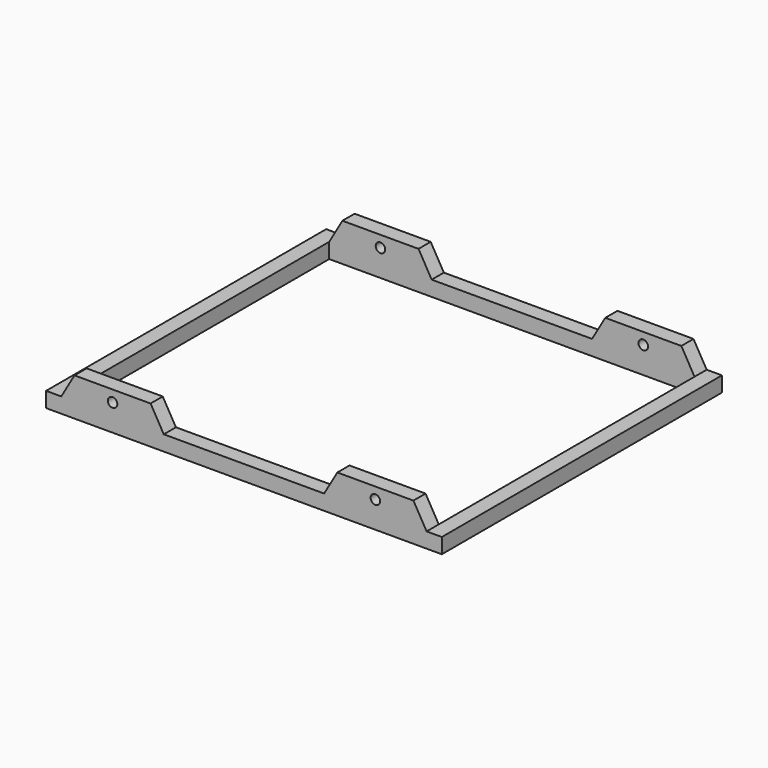
from build123d import *

# Parameters (mm, degrees)
F1_W     = 25.4
F1_H     = 25.4
F4_DEPTH = 25.4
F5_D     = 15.875


with BuildPart() as f2:
    # F2: sweep along a path in F0
    with BuildLine(Plane.XY) as f2_path:
        Line((-304.8, -266.75), (-304.8, 266.75))
        Line((-304.8, 266.75), (304.8, 266.75))
        Line((304.8, 266.75), (304.8, -266.75))
        Line((304.8, -266.75), (-304.8, -266.75))
    # F1 (on Front) → F2 (sweep)
    with BuildSketch(Plane.XZ):
        with Locations((-317.5, 0)):
            Rectangle(F1_W, F1_H)
    sweep(path=f2_path.line, transition=Transition.RIGHT)

    # F3 (on face) → F4 (join, through all)
    with BuildSketch(Plane.XZ.offset(292.15)):
        Polygon((133.8059094878, 12.7), (304.8, 12.7), (282.8029547439, 50.8), (155.8029547439, 50.8), align=None)
    extrude(amount=-F4_DEPTH)

    # F5 (through all)
    with Locations(Plane.XZ.offset(292.15)):
        with Locations((219.3029547439, 31.7)):
            Hole(F5_D / 2)


with BuildPart() as f6_1:
    # F6: instance of F2
    add(f2.part.mirror(Plane.YZ))


with BuildPart() as f2_1:
    add(f2.part)

    add(f6_1.part)  # F7 merges F6_1
    # F7: F6_1, F2 across plane
    add(f6_1.part.mirror(Plane.XZ))
    add(f2.part.mirror(Plane.XZ))


solid = f2_1.part
